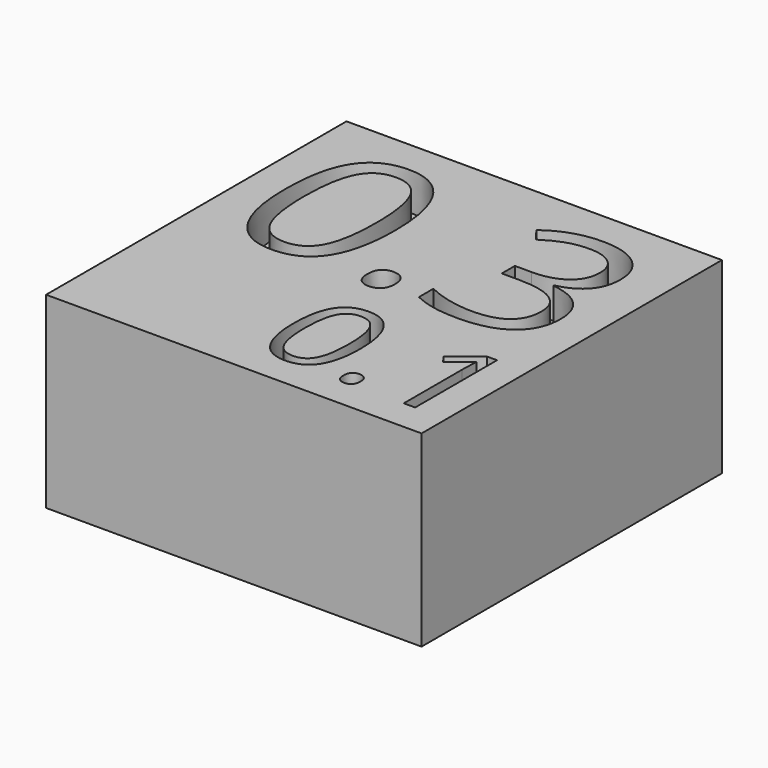
from build123d import *

# Parameters (mm, degrees)
F0_W           = 10
F0_H           = 10
F1_DEPTH       = 5
F2_TEXT_SIZE   = 6.25
F2_TEXT_SIZE_2 = 3.8194444444
F3_DEPTH       = 1


# Not quite as in the source:
# - a feature names something its author has since deleted; it is built from what else it names
# - Text() gives the source's letters only with a copy of the font that has no kerning and outlines rounded to 1/6400 em; it was checked with that copy


with BuildPart() as f1:
    # F0 (on Top) → F1 (new body)
    with BuildSketch(Plane.XY):
        Rectangle(F0_W, F0_H)
    extrude(amount=F1_DEPTH)

    # F2 (on face) → F3 (cut)
    with BuildSketch(Plane.XY.offset(5)):
        with Locations((-4.4020166787, -0.4192900058)):
            Text('0.3', F2_TEXT_SIZE, font='Open Sans', text_align=(TextAlign.LEFT, TextAlign.BOTTOM))
        with Locations((-0.3668521055, -4.1716412553)):
            Text('0.1', F2_TEXT_SIZE_2, font='Open Sans', text_align=(TextAlign.LEFT, TextAlign.BOTTOM))
    extrude(amount=-F3_DEPTH, mode=Mode.SUBTRACT)


solid = f1.part
